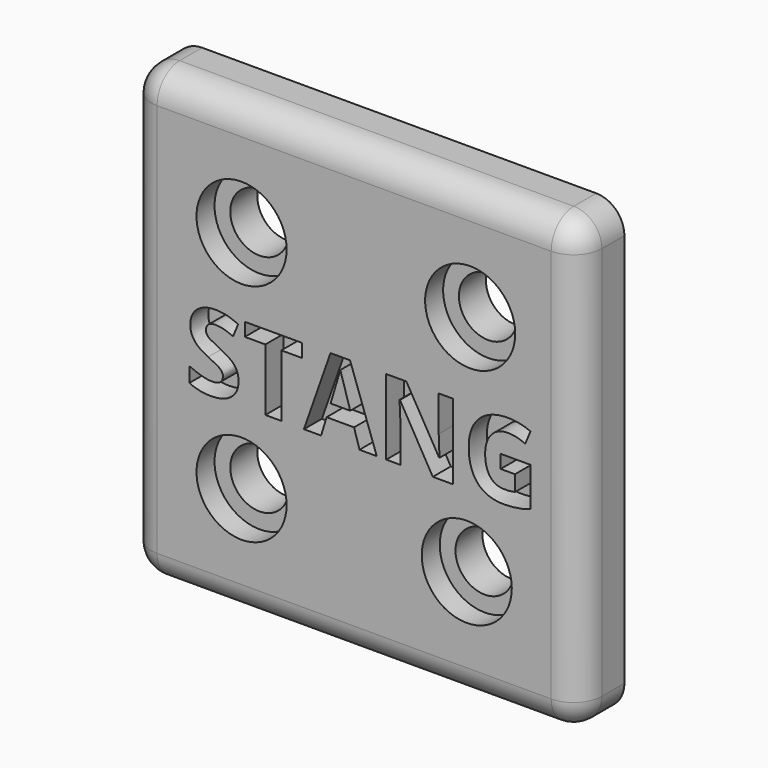
from build123d import *

# Parameters (mm, degrees)
F0_W           = 50.8
F0_H           = 50.8
F2_DEPTH       = 6.35
F3_D           = 6.604
F3_CBORE_D     = 10.16
F3_CBORE_DEPTH = 2.54
F4_R           = 3.175
F5_R           = 3.175
F6_TEXT_SIZE   = 11.9091140934
F7_DEPTH       = 2.54


# Not quite as in the source:
# - Text() gives the source's letters only with a copy of the font that has no kerning and outlines rounded to 1/6400 em; it was checked with that copy


with BuildPart() as f2:
    # F0 (on Front) → F2 (new body)
    with BuildSketch(Plane.XZ):
        Rectangle(F0_W, F0_H)
    extrude(amount=-F2_DEPTH)

    # F3 (through all)
    with Locations(Plane.XZ):
        with Locations((-12.7, 12.7), (13.0855841562, 12.7), (12.7, -12.7), (-12.7, -12.7)):
            CounterBoreHole(F3_D / 2, F3_CBORE_D / 2, F3_CBORE_DEPTH)

    # F4
    f4_edges = [f2.edges().sort_by_distance(p)[0] for p in [
        (25.4, 3.175, 25.4),
        (25.4, 3.175, -25.4),
        (-25.4, 3.175, -25.4),
        (-25.4, 3.175, 25.4),
    ]]
    fillet(f4_edges, radius=F4_R)

    # F5
    f5_edges = [f2.edges().sort_by_distance(p)[0] for p in [
        (0, 0, 25.4),
    ]]
    fillet(f5_edges, radius=F5_R)

    # F6 (on Front) → F7 (cut)
    with BuildSketch(Plane.XZ):
        with Locations((-19.1244727466, -4.5165796764)):
            Text('STANG', F6_TEXT_SIZE, font='Open Sans', font_style=FontStyle.BOLD, text_align=(TextAlign.LEFT, TextAlign.BOTTOM))
    extrude(amount=-F7_DEPTH, mode=Mode.SUBTRACT)


solid = f2.part
